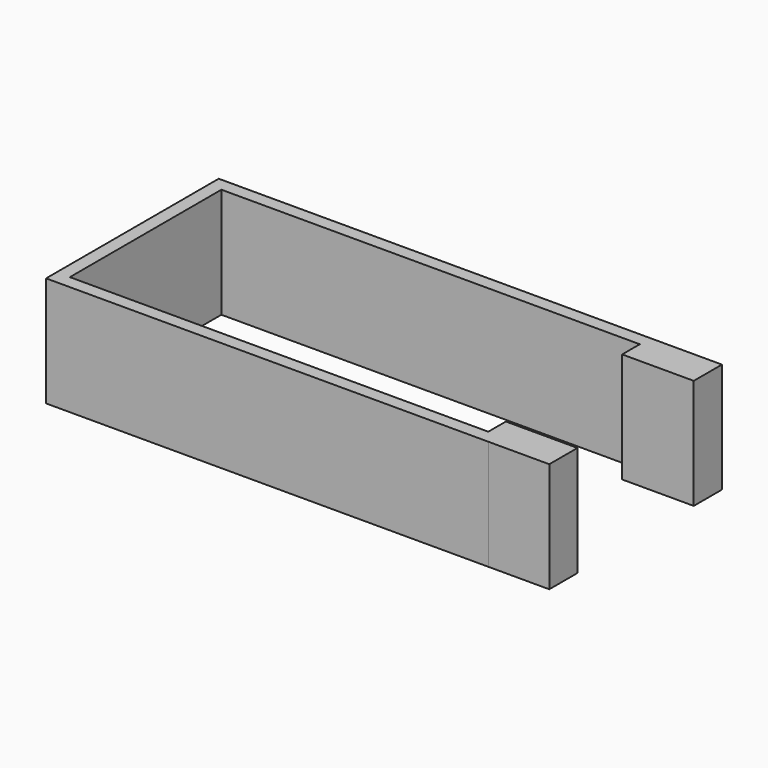
from build123d import *

# Parameters (mm, degrees)
F0_W     = 6.5
F0_H     = 2
F1_DEPTH = 10


# Not quite as in the source:
# - ends of sketch curves that miss each other by under 0.0002 mm in the source are joined


with BuildPart() as f1:
    # F0 (on Top) → F1 (new body)
    with BuildSketch(Plane.XY):
        Polygon((-44.5, -8.6), (-44.5, 0), (-44.5, 8.6), (-6.5, 8.6), (0, 8.6), (0, 9.8000001162), (-5.5, 9.8000001162), (-45.7, 9.8), (-45.7, 0), (-45.7, -9.8), (-5.5, -9.8), (0, -9.8000001162), (0, -8.6), (0, -6.6), (-6.5, -6.6), (-6.5, -8.6), align=None)
        with Locations((-3.25, 7.6)):
            Rectangle(F0_W, F0_H)
    extrude(amount=F1_DEPTH)


solid = f1.part
